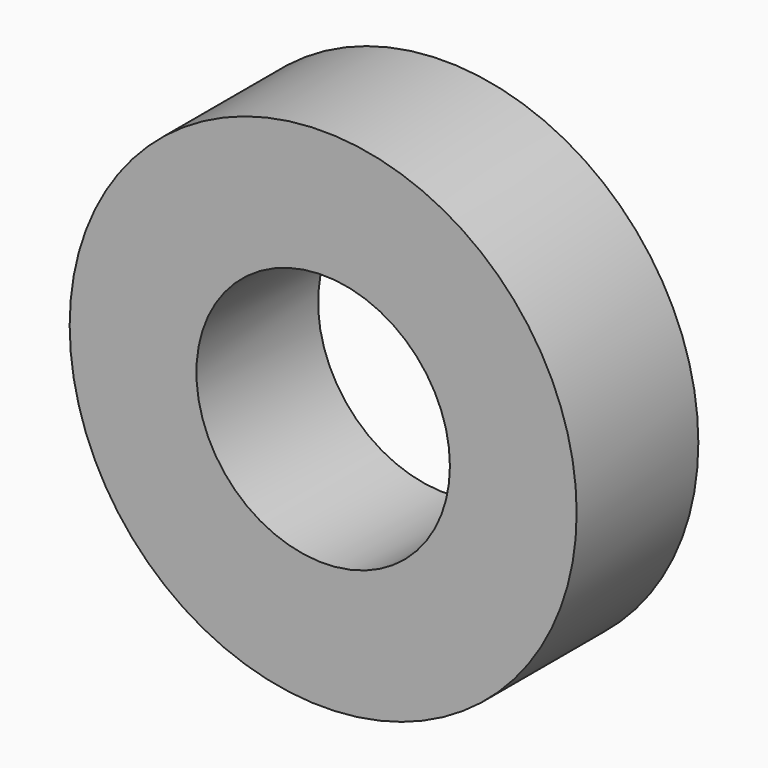
from build123d import *

# Parameters (mm, degrees)
F0_R     = 16
F0_R_2   = 8
F1_DEPTH = 9.6


# Not quite as in the source:
# - a feature names something its author has since deleted; it is built from what else it names


with BuildPart() as f1:
    # F0 (on Front) → F1 (new body)
    with BuildSketch(Plane.XZ):
        Circle(F0_R)
        Circle(F0_R_2, mode=Mode.SUBTRACT)
    extrude(amount=F1_DEPTH)


solid = f1.part
